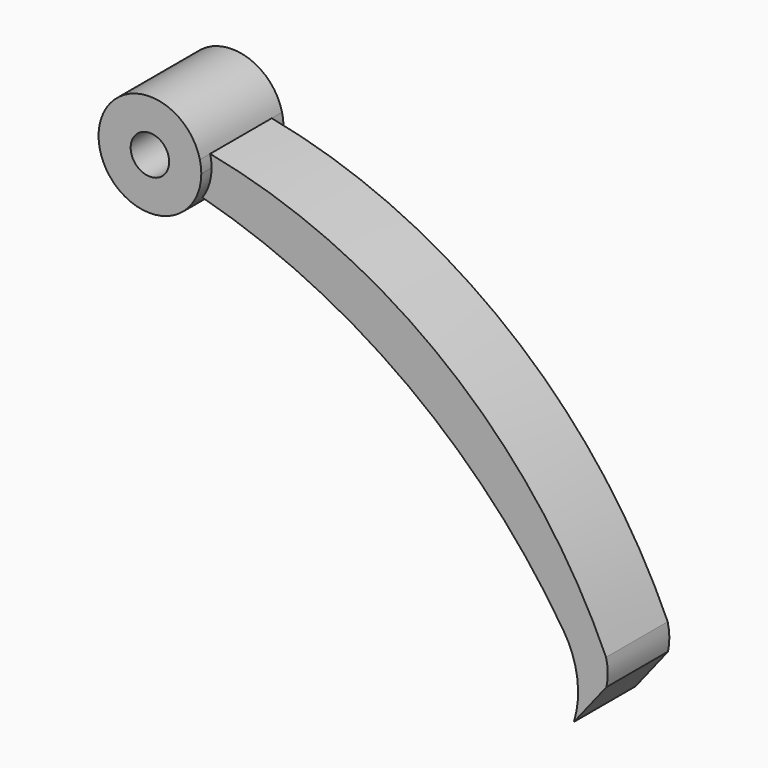
from build123d import *

# Parameters (mm, degrees)
F1_DEPTH = 3
F0_R     = 1.5
F2_DEPTH = 4


with BuildPart() as f1:
    # F0 (on Front) → F1 (new body, symmetric)
    with BuildSketch(Plane.XZ):
        with BuildLine():
            ThreePointArc((3.29609, 67.379701), (19.254375, 59.728993), (31.399545, 46.856734))
            ThreePointArc((31.399545, 46.856734), (32.484161, 43.93561), (32.219696, 40.830868))
            Line((32.219696, 40.830868), (34.755978, 44.04202))
            ThreePointArc((34.755978, 44.04202), (34.85532, 45.062099), (34.729093, 46.079202))
            ThreePointArc((34.729093, 46.079202), (22.301334, 62.092348), (3.890979, 70.573441))
            ThreePointArc((3.890979, 70.573441), (3.972651, 70.112878), (4, 69.645929))
            ThreePointArc((4, 69.645929), (3.819971, 68.459414), (3.29609, 67.379701))
        make_face()
    extrude(amount=F1_DEPTH, both=True)

    # F0 (on Front) → F2 (join, symmetric)
    with BuildSketch(Plane.XZ):
        with BuildLine():
            ThreePointArc((3.890979, 70.573441), (-3.932364, 70.3784), (3.29609, 67.379701))
            ThreePointArc((3.29609, 67.379701), (3.819971, 68.459414), (4, 69.645929))
            ThreePointArc((4, 69.645929), (3.972651, 70.112878), (3.890979, 70.573441))
        make_face()
        with Locations((0, 69.645929)):
            Circle(F0_R, mode=Mode.SUBTRACT)
    extrude(amount=F2_DEPTH, both=True)


solid = f1.part
